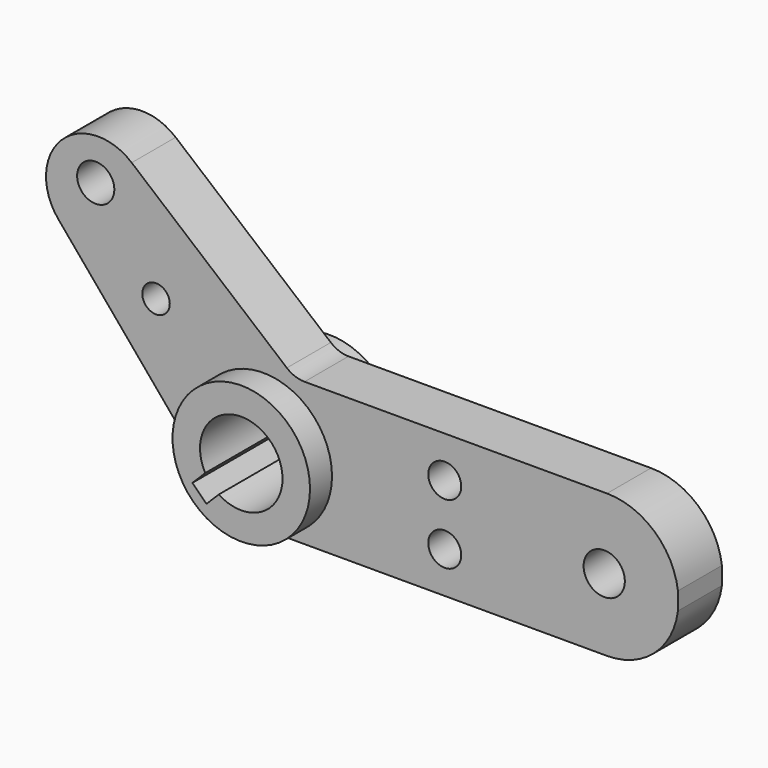
from build123d import *

# Parameters (mm, degrees)
F1_DEPTH      = 12.7
F2_R          = 15.875
F2_R_2        = 9.525
F3_DEPTH      = 6.35
F3_DEPTH_BACK = 19.05
F4_R          = 9.525
F5_DEPTH      = 25.4
F7_DEPTH      = 25.401
F8_R          = 4.7625
F8_R_2        = 3.81
F8_R_3        = 3.175
F8_R_4        = 4.2961277226
F9_DEPTH      = 19.051
F12_DEPTH     = 19.051
F14_DEPTH     = 25.4


# Not quite as in the source:
# - after a boolean that leaves OpenCascade's solid faulty, fix() repairs it


with BuildPart() as f1:
    # F0 (on Front) → F1 (new body)
    with BuildSketch(Plane.XZ):
        with BuildLine():
            ThreePointArc((-12.1609555345, 5.6707466962), (-6.7090649051, 1.4873638808), (0, 0))
            Line((0, 0), (79.375, 0))
            ThreePointArc((79.375, 0), (95.885, 16.51), (79.375, 33.02))
            Line((79.375, 33.02), (9.525, 33.02))
            ThreePointArc((9.525, 33.02), (7.3531720899, 33.402951858), (5.4432986785, 34.5056177862))
            Line((5.4432986785, 34.5056177862), (-30.3843620081, 64.5685946542))
            ThreePointArc((-30.3843620081, 64.5685946542), (-46.6383026366, 63.8589322804), (-47.3479650105, 47.6049916518))
            Line((-47.3479650105, 47.6049916518), (-12.1609555345, 5.6707466962))
        make_face()
    extrude(amount=F1_DEPTH)

    # F2 (on face) → F3 (join, two sides)
    with BuildSketch(Plane.XZ.offset(12.7)) as f3_sk:
        with Locations((0, 15.875)):
            Circle(F2_R)
        with Locations((0, 15.875)):
            Circle(F2_R_2, mode=Mode.SUBTRACT)
    extrude(amount=F3_DEPTH)
    extrude(f3_sk.sketch, amount=-F3_DEPTH_BACK)

    add(f1.part.fix(), mode=Mode.REPLACE)

    # F4 (on face) → F5 (cut)
    with BuildSketch(Plane.XZ.offset(12.7)):
        with Locations((0, 15.875)):
            Circle(F4_R)
    extrude(amount=-F5_DEPTH, mode=Mode.SUBTRACT)

    # F6 (on face) → F7 (cut, through all)
    with BuildSketch(Plane.XZ.offset(19.05)):
        with BuildLine():
            Line((-8.3178005381, 11.2338989228), (-11.2676186575, 8.2840808033))
            Line((-11.2676186575, 8.2840808033), (-8.034726454, 5.0511885997))
            Line((-8.034726454, 5.0511885997), (-5.1946960102, 7.8912190435))
            ThreePointArc((-5.1946960102, 7.8912190435), (-6.959904305, 9.3722807946), (-8.3178005381, 11.2338989228))
        make_face()
    extrude(amount=-F7_DEPTH, mode=Mode.SUBTRACT)

    # F8 (on face) → F9 (cut, through all)
    with BuildSketch(Plane.XZ.offset(12.7)):
        with Locations((78.74, 16.51)):
            Circle(F8_R)
        with Locations((41.91, 23.495)):
            Circle(F8_R_2)
        with Locations((41.91, 9.525)):
            Circle(F8_R_2)
        with Locations((-24.765, 38.735)):
            Circle(F8_R_3)
        with Locations((-38.6896171983, 57.7962485902)):
            Circle(F8_R_4)
    extrude(amount=-F9_DEPTH, mode=Mode.SUBTRACT)

    # F11 (on face) → F12 (cut, through all)
    with BuildSketch(Plane.XZ.offset(12.7)):
        with BuildLine():
            Line((95.758, 18.5538715713), (95.758, 14.4661284287))
            ThreePointArc((95.758, 14.4661284287), (95.885, 16.51), (95.758, 18.5538715713))
        make_face()
        with BuildLine():
            ThreePointArc((95.758, 18.5538715713), (95.885, 16.51), (95.758, 14.4661284287))
            Line((95.758, 14.4661284287), (95.758, 13.97))
            Line((95.758, 13.97), (97.3146509769, 13.97))
            Line((97.3146509769, 13.97), (97.3146509769, 19.05))
            Line((97.3146509769, 19.05), (95.758, 19.05))
            Line((95.758, 19.05), (95.758, 18.5538715713))
        make_face()
    extrude(amount=-F12_DEPTH, mode=Mode.SUBTRACT)

    # F13 (on face) → F14 (join)
    with BuildSketch(Plane.XZ.offset(19.05)):
        with BuildLine():
            Line((5.9313747803, 23.3278127721), (7.0446438565, 22.2858203792))
            ThreePointArc((7.0446438565, 22.2858203792), (6.5088940652, 22.8291299274), (5.9313747803, 23.3278127721))
        make_face()
    extrude(amount=-F14_DEPTH)


solid = f1.part
